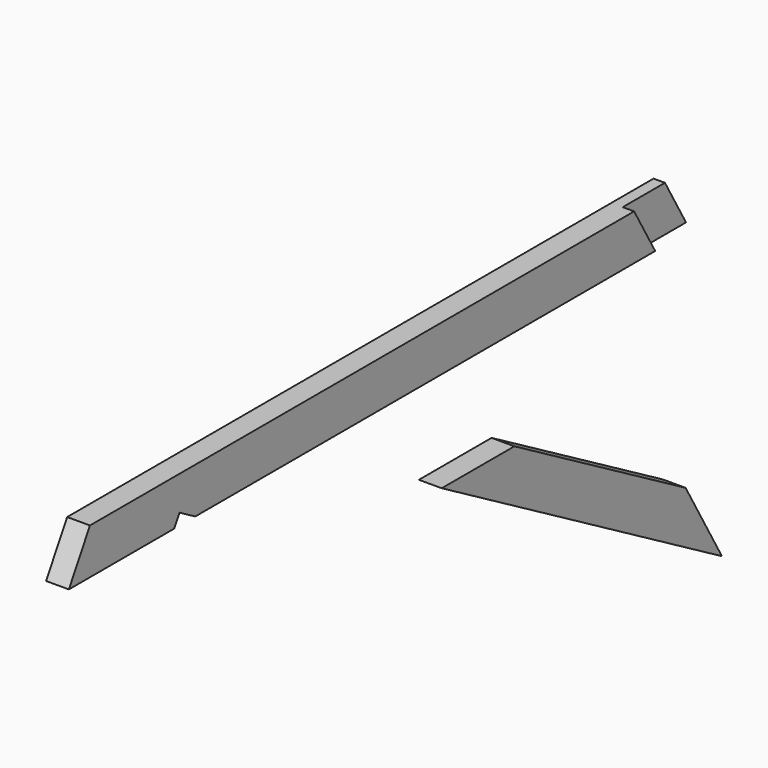
from build123d import *

# Parameters (mm, degrees)
F1_DEPTH = 60
F2_DEPTH = 30
F5_DEPTH = 60


with BuildPart() as f1:
    # F0 (on Right) → F1 (new body)
    with BuildSketch(Plane.YZ):
        Polygon((-2144.0138730987, -709.7315810384), (-2213.2959054015, -829.7315810384), (-1866.9698524821, -829.7315810384), (-1849.6493444064, -799.7315810384), (-1797.6878201794, -829.7315810384), (-285.3045596479, -829.7315810384), (-354.5865919507, -709.7315810384), align=None)
    extrude(amount=F1_DEPTH)

    # F0 (on Right) → F2 (join)
    with BuildSketch(Plane.YZ):
        Polygon((-215.7480825998, -709.7315810384), (-354.5865919507, -709.7315810384), (-285.3045596479, -829.7315810384), (-146.466050297, -829.7315810384), align=None)
    extrude(amount=F2_DEPTH)


with BuildPart() as f5:
    # F3 (on Right) → F5 (new body)
    with BuildSketch(Plane.YZ):
        Polygon((-185.3331125225, -1418.8327086396), (-466.878688753, -1256.2822944138), (-748.4242649835, -1093.731880188), (-987.3136878014, -1093.731880188), (-526.6010444575, -1359.7244488417), (-65.8884011135, -1625.7170174953), align=None)
    extrude(amount=F5_DEPTH)


solid = Compound([f1.part, f5.part])
